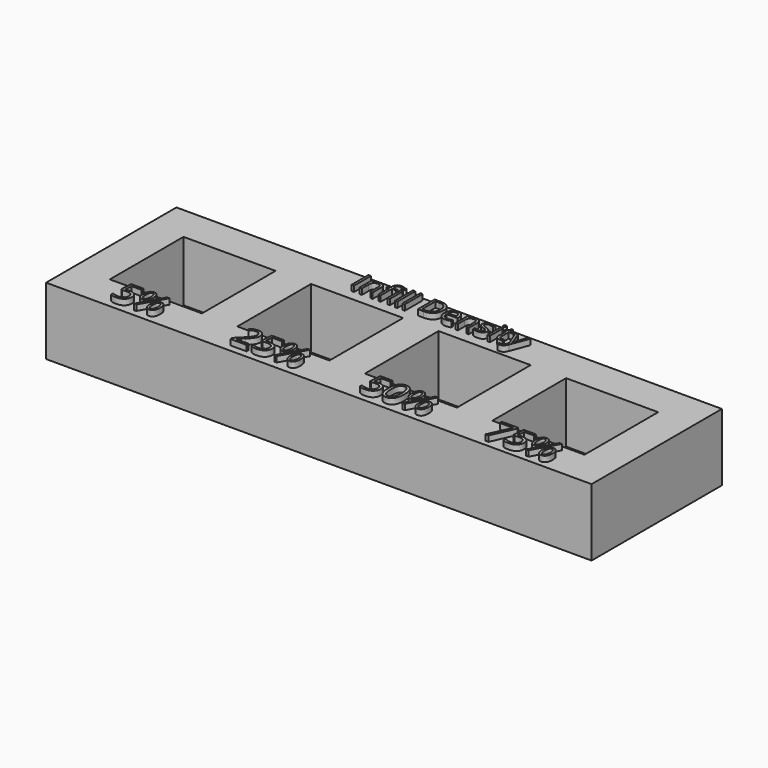
from build123d import *

# Parameters (mm, degrees)
F0_W           = 154
F0_H           = 46
F0_W_2         = 26
F0_H_2         = 26
F1_DEPTH       = 19
F2_DEPTH       = 17
F3_TEXT_SIZE   = 8.3107346048
F3_TEXT_SIZE_2 = 9.7222222222
F4_DEPTH       = 1.6


# Not quite as in the source:
# - Text() gives the source's letters only with a copy of the font that has no kerning and outlines rounded to 1/6400 em; it was checked with that copy


with BuildPart() as f1:
    # F0 (on Top) → F1 (new body)
    with BuildSketch(Plane.XY):
        with Locations((-77, 23)):
            Rectangle(F0_W, F0_H)
        with Locations((-131, 23)):
            Rectangle(F0_W_2, F0_H_2, mode=Mode.SUBTRACT)
        with Locations((-95, 23)):
            Rectangle(F0_W_2, F0_H_2, mode=Mode.SUBTRACT)
        with Locations((-59, 23)):
            Rectangle(F0_W_2, F0_H_2, mode=Mode.SUBTRACT)
        with Locations((-23, 23)):
            Rectangle(F0_W_2, F0_H_2, mode=Mode.SUBTRACT)
        with Locations((-131, 23)):
            Rectangle(F0_W_2, F0_H_2)
        with Locations((-95, 23)):
            Rectangle(F0_W_2, F0_H_2)
        with Locations((-59, 23)):
            Rectangle(F0_W_2, F0_H_2)
        with Locations((-23, 23)):
            Rectangle(F0_W_2, F0_H_2)
    extrude(amount=-F1_DEPTH)

    # F0 (on Top) → F2 (cut)
    with BuildSketch(Plane.XY):
        with Locations((-131, 23)):
            Rectangle(F0_W_2, F0_H_2)
        with Locations((-95, 23)):
            Rectangle(F0_W_2, F0_H_2)
        with Locations((-59, 23)):
            Rectangle(F0_W_2, F0_H_2)
        with Locations((-23, 23)):
            Rectangle(F0_W_2, F0_H_2)
    extrude(amount=-F2_DEPTH, mode=Mode.SUBTRACT)

    # F3 (on face) → F4 (join)
    with BuildSketch(Plane.XY):
        with Locations((-99.680736661, 38.9110893011)):
            Text('Infill Density', F3_TEXT_SIZE, font='Open Sans', text_align=(TextAlign.LEFT, TextAlign.BOTTOM))
        with Locations((-138.0017995834, 1.8431187905)):
            Text('5%', F3_TEXT_SIZE_2, font='Open Sans', text_align=(TextAlign.LEFT, TextAlign.BOTTOM))
        with Locations((-104.0181741118, 1.9840670116)):
            Text('25%', F3_TEXT_SIZE_2, font='Open Sans', text_align=(TextAlign.LEFT, TextAlign.BOTTOM))
        with Locations((-67.736055702, 1.8439807296)):
            Text('50%', F3_TEXT_SIZE_2, font='Open Sans', text_align=(TextAlign.LEFT, TextAlign.BOTTOM))
        with Locations((-32.5746238232, 1.5638100281)):
            Text('75%', F3_TEXT_SIZE_2, font='Open Sans', text_align=(TextAlign.LEFT, TextAlign.BOTTOM))
    extrude(amount=F4_DEPTH)


solid = f1.part
